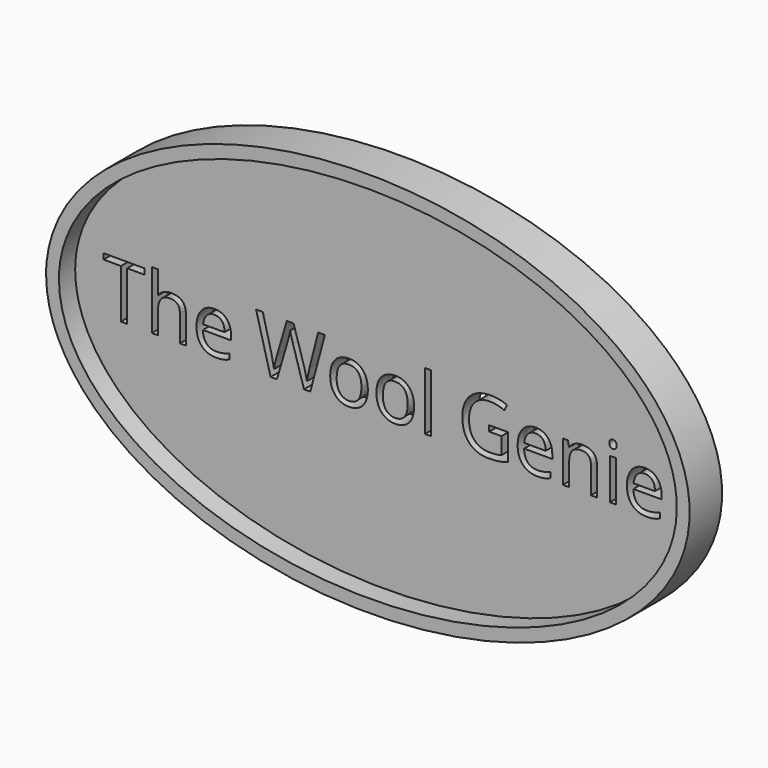
from build123d import *

# Parameters (mm, degrees)
F1_DEPTH     = 4
F3_DEPTH     = 2
F4_TEXT_SIZE = 7.5519967779
F5_DEPTH     = 2.54


# Not quite as in the source:
# - Text() gives the source's letters only with a copy of the font that has no kerning and outlines rounded to 1/6400 em; it was checked with that copy


with BuildPart() as f1:
    # F0 (on Front) → F1 (new body)
    with BuildSketch(Plane.XZ):
        with BuildLine():
            add(Edge.make_bspline(
                [(-31.75, 0), (-31.75, -32.9955678842), (15.875, -16.4977839421), (63.5, 0), (15.875, 16.4977839421), (-31.75, 32.9955678842), (-31.75, 0)],
                knots=[0, 0, 0, 2.0943951024, 2.0943951024, 4.1887902048, 4.1887902048, 6.2831853072, 6.2831853072, 6.2831853072], degree=2, weights=[1, 0.5, 1, 0.5, 1, 0.5, 1]))
        make_face()
    extrude(amount=F1_DEPTH)

    # F2 (on face) → F3 (cut)
    with BuildSketch(Plane.XZ.offset(4)):
        with BuildLine():
            add(Edge.make_bspline(
                [(-30.48, 0), (-30.48, -30.7958633586), (15.24, -15.3979316793), (60.96, 0), (15.24, 15.3979316793), (-30.48, 30.7958633586), (-30.48, 0)],
                knots=[0, 0, 0, 2.0943951024, 2.0943951024, 4.1887902048, 4.1887902048, 6.2831853072, 6.2831853072, 6.2831853072], degree=2, weights=[1, 0.5, 1, 0.5, 1, 0.5, 1]))
        make_face()
    extrude(amount=-F3_DEPTH, mode=Mode.SUBTRACT)

    # F4 (on face) → F5 (cut)
    with BuildSketch(Plane.XZ.offset(2)):
        with Locations((-27.7441835886, -3.0305724672)):
            Text('The Wool Genie', F4_TEXT_SIZE, font='Open Sans', text_align=(TextAlign.LEFT, TextAlign.BOTTOM))
    extrude(amount=-F5_DEPTH, mode=Mode.SUBTRACT)


solid = f1.part
